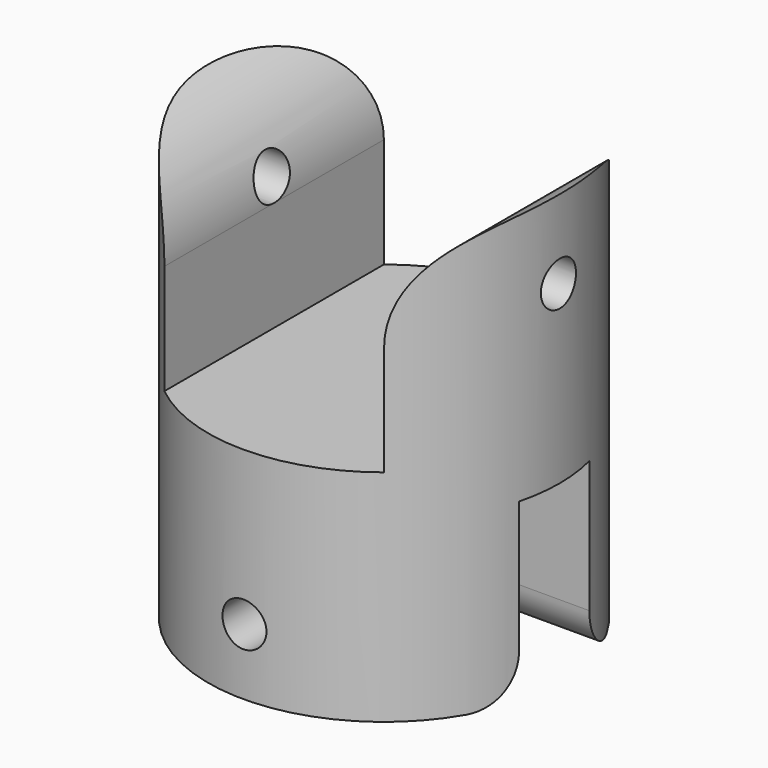
from build123d import *

# Parameters (mm, degrees)
F0_R         = 8
F1_DEPTH     = 20
F2_W         = 10
F2_H         = 16
F3_DEPTH     = 10
F4_W         = 16
F4_H         = 4
F5_DEPTH     = 8
F6_R         = 1
F7_DEPTH     = 8
F8_R         = 1
F9_DEPTH     = 8
F10_T1_DEPTH = 37.4899959968
F11_R        = 2


# Not quite as in the source:
# - a fillet or chamfer that OpenCascade refuses, or shapes differently, is made with other operations: its cross-section is extruded or revolved along the edge and cut away or added


with BuildPart() as f1:
    # F0 (on Top) → F1 (new body)
    with BuildSketch(Plane.XY):
        Circle(F0_R)
    extrude(amount=F1_DEPTH)

    # F2 (on face) → F3 (cut)
    with BuildSketch(Plane.XY.offset(20)):
        Rectangle(F2_W, F2_H)
    extrude(amount=-F3_DEPTH, mode=Mode.SUBTRACT)

    # F4 (on face) → F5 (cut)
    with BuildSketch(Plane(origin=(0, 0, 0), x_dir=(1, 0, 0), z_dir=(0, 0, -1))):
        Rectangle(F4_W, F4_H)
    extrude(amount=-F5_DEPTH, mode=Mode.SUBTRACT)

    # F6 (on Right) → F7 (cut, symmetric)
    with BuildSketch(Plane.YZ):
        with Locations((0, 16)):
            Circle(F6_R)
    extrude(amount=F7_DEPTH, both=True, mode=Mode.SUBTRACT)

    # F8 (on Front) → F9 (cut, symmetric)
    with BuildSketch(Plane.XZ):
        with Locations((0, 3)):
            Circle(F8_R)
    extrude(amount=F9_DEPTH, both=True, mode=Mode.SUBTRACT)

    # F10: fillet of radius 5 on 2 edges, made by hand

    # F10_s2 → F10_t1 (cut)
    with BuildSketch(Plane.XZ.offset(-18.7449979984)):
        with BuildLine():
            ThreePointArc((-10, 20), (-6.4644660941, 18.5355339059), (-5, 15))
            Line((-5, 15), (-5, 20))
            Line((-5, 20), (-10, 20))
        make_face()
        with BuildLine():
            ThreePointArc((5, 15), (6.4644660941, 18.5355339059), (10, 20))
            Line((10, 20), (5, 20))
            Line((5, 20), (5, 15))
        make_face()
    extrude(amount=F10_T1_DEPTH, mode=Mode.SUBTRACT)

    # F11
    f11_edges = [f1.edges().sort_by_distance(p)[0] for p in [
        (0, -2, 0),
        (0, 2, 0),
    ]]
    fillet(f11_edges, radius=F11_R)


solid = f1.part
